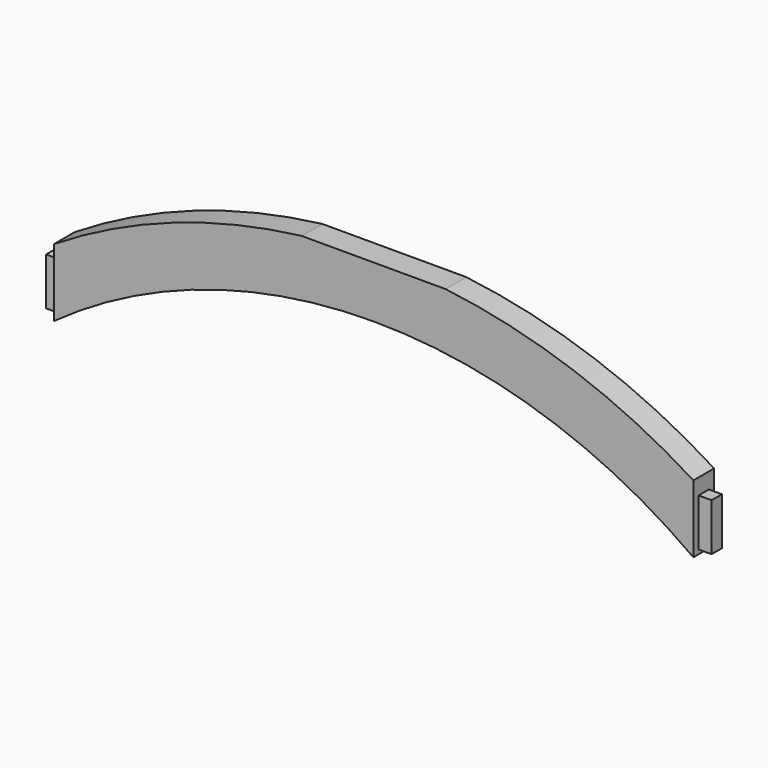
from build123d import *

# Parameters (mm, degrees)
F1_DEPTH = 38.1
F2_W     = 19.05
F2_H     = 69.85
F3_DEPTH = 19.05


# Not quite as in the source:
# - a pattern or mirror of a feature is missing from the dataset's text; its kind, count and spacing are read off the source's solid


with BuildPart() as f1:
    # F0 (on Front) → F1 (new body)
    with BuildSketch(Plane.XZ):
        with BuildLine():
            ThreePointArc((25.4, 147.32), (495.3, 299.72), (965.2, 147.32))
            Line((965.2, 147.32), (965.2, 246.8872163374))
            ThreePointArc((965.2, 246.8872163374), (790.2509366907, 331.5626859382), (601.016852567, 375.92))
            Line((601.016852567, 375.92), (389.583147433, 375.92))
            ThreePointArc((389.583147433, 375.92), (200.3490633093, 331.5626859382), (25.4, 246.8872163374))
            Line((25.4, 246.8872163374), (25.4, 217.17))
            Line((25.4, 217.17), (25.4, 153.67))
            Line((25.4, 153.67), (25.4, 147.32))
        make_face()
    extrude(amount=F1_DEPTH)

    # F2 (on face) → F3 (join)
    with BuildSketch(Plane.YZ.offset(965.2)):
        with Locations((-19.05, 188.595)):
            Rectangle(F2_W, F2_H)
    f3 = extrude(amount=F3_DEPTH)

    # F3_copies: F3 across plane
    add(f3.mirror(Plane(origin=(495.3, 0, 0), x_dir=(0, 0, -1), z_dir=(-1, 0, 0))))


solid = f1.part
